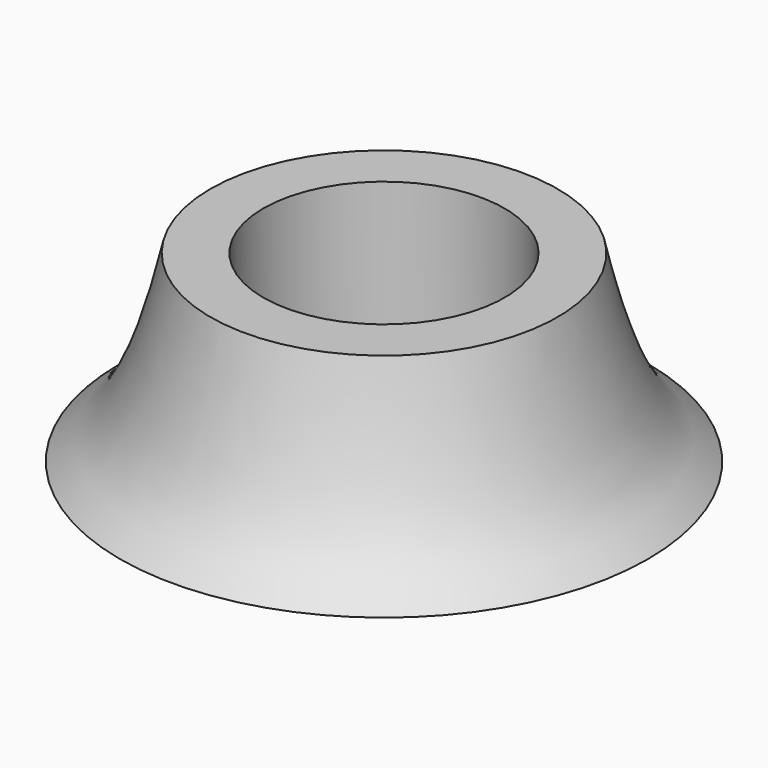
from build123d import *


with BuildPart() as f1:
    # F0 (on Front) → F1 (revolve)
    with BuildSketch(Plane.XZ):
        with BuildLine():
            Line((-3.175, 0), (-3.175, 4.826))
            Line((-3.175, 4.826), (-4.5654736459, 4.826))
            add(Edge.make_bspline(
                [(-4.5654736459, 4.826), (-4.8888199963, 3.3683741931), (-5.5216582711, 1.3934291844), (-6.2301136902, 0.564768836), (-6.9453125, 0)],
                knots=[0, 0, 0, 0, 0.5708708677, 1, 1, 1, 1], degree=3))
            Line((-6.9453125, 0), (-5.2552358247, 0))
            Line((-5.2552358247, 0), (-4.8580123112, 0.467726466))
            Line((-4.8580123112, 0.467726466), (-4.0218508802, 0.467726466))
            Line((-4.0218508802, 0.467726466), (-4.0218508802, 0))
            Line((-4.0218508802, 0), (-3.175, 0))
        make_face()
    revolve(axis=Axis((0, 0, 4.2204221714), (0, 0, 1)))


solid = f1.part
